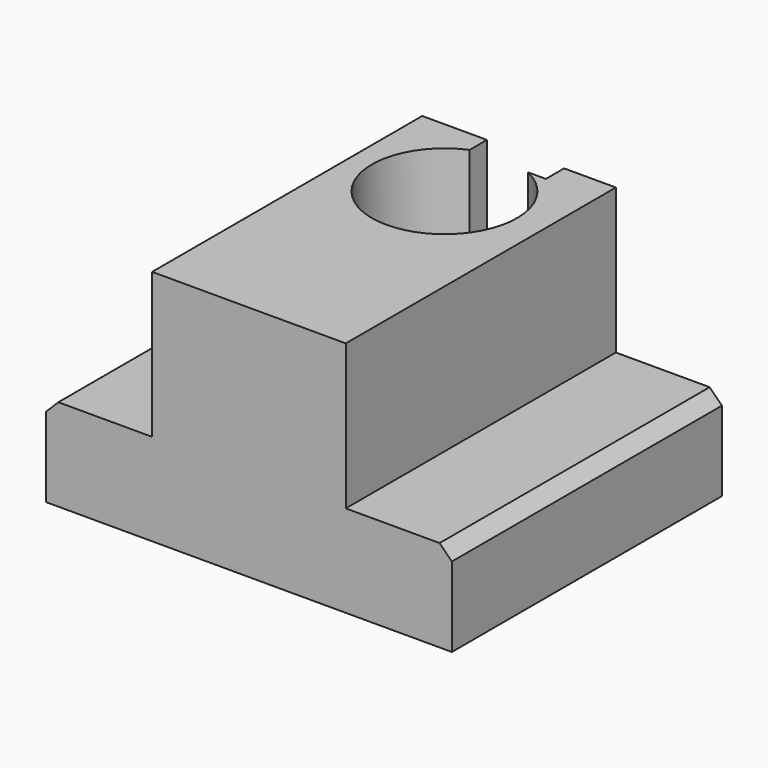
from build123d import *

# Parameters (mm, degrees)
F1_DEPTH = 35.0012
F2_R     = 7.5311
F3_DEPTH = 24.638
F4_DEPTH = 15.0622
F5_W     = 7.9995468259
F5_H     = 14.370085096
F6_DEPTH = 2.3622
F7_SIZE  = 1.27


# Not quite as in the source:
# - a feature names something its author has since deleted; it is built from what else it names


with BuildPart() as f1:
    # F0 (on Front) → F1 (new body)
    with BuildSketch(Plane.XZ):
        Polygon((-22.2087535855, 0), (-22.0162163296, 0), (19.8619475364, 0), (19.8619475364, 9.5335517829), (8.8637475364, 9.5335517829), (8.8637475364, 24.5957517829), (-11.2105535855, 24.5957517829), (-11.2105535855, 9.5335517829), (-22.2087535855, 9.5335517829), align=None)
    extrude(amount=F1_DEPTH)

    # F2 (on Top) → F3 (cut)
    with BuildSketch(Plane.XY):
        with Locations((-1.5582955675, -9.1819977388)):
            Circle(F2_R)
    extrude(amount=F3_DEPTH, mode=Mode.SUBTRACT)

    # F2 (on Top) → F4 (join)
    with BuildSketch(Plane.XY):
        with Locations((-1.5582955675, -9.1819977388)):
            Circle(F2_R)
    extrude(amount=F4_DEPTH)

    # F5 (on face) → F6 (cut, symmetric)
    with BuildSketch(Plane.XZ):
        with Locations((-0.500776805, 17.4107092349)):
            Rectangle(F5_W, F5_H)
    extrude(amount=F6_DEPTH, both=True, mode=Mode.SUBTRACT)

    # F7
    f7_edges = [f1.edges().sort_by_distance(p)[0] for p in [
        (19.861948, -17.5006, 9.533552),
        (-22.208754, -17.5006, 9.533552),
    ]]
    chamfer(f7_edges, length=F7_SIZE)


solid = f1.part
